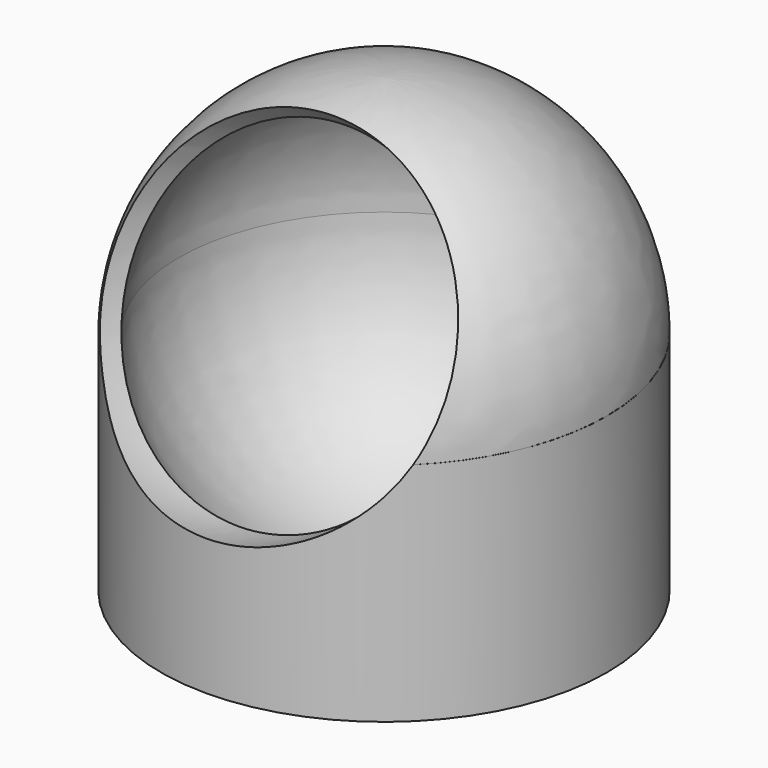
from build123d import *

# Parameters (mm, degrees)
F4_R     = 25.2
F7_DEPTH = 25.4980942398


with BuildPart() as f2:
    # F1 (on Front) → F2 (revolve)
    with BuildSketch(Plane.XZ):
        with BuildLine():
            ThreePointArc((0, 0), (17.8293562003, 7.5774317225), (25.1882466714, 25.4980942398))
            ThreePointArc((25.1882466714, 25.4980942398), (17.8293562003, 43.4187567571), (0, 50.9961884796))
            Line((0, 50.9961884796), (0, 48.9960262735))
            ThreePointArc((0, 48.9960262735), (16.4151143283, 42.0045141541), (23.1882466714, 25.4980942398))
            ThreePointArc((23.1882466714, 25.4980942398), (16.4151143283, 8.9916743255), (0, 2.0001622061))
            Line((0, 2.0001622061), (0, 0))
        make_face()
        with BuildLine():
            ThreePointArc((23.1882466714, 25.4980942398), (16.4151143283, 42.0045141541), (0, 48.9960262735))
            Line((0, 48.9960262735), (0, 2.0001622061))
            ThreePointArc((0, 2.0001622061), (16.4151143283, 8.9916743255), (23.1882466714, 25.4980942398))
        make_face()
    revolve(axis=Axis((0, 0, 25.4980942398), (0, 0, -1)))

    # F4 (on Top) → F7 (join, through all)
    with BuildSketch(Plane.XY):
        Circle(F4_R)
    extrude(amount=F7_DEPTH)


with BuildPart() as f3:
    # F1 (on Front) → F3 (revolve)
    with BuildSketch(Plane.XZ):
        with BuildLine():
            ThreePointArc((23.1882466714, 25.4980942398), (16.4151143283, 42.0045141541), (0, 48.9960262735))
            Line((0, 48.9960262735), (0, 2.0001622061))
            ThreePointArc((0, 2.0001622061), (16.4151143283, 8.9916743255), (23.1882466714, 25.4980942398))
        make_face()
    revolve(axis=Axis((0, 0, 25.4980942398), (0, 0, -1)))


with BuildPart() as f9:
    # F8 (on Right) → F9 (revolve)
    with BuildSketch(Plane.YZ):
        with BuildLine():
            Line((-19.8910422623, 14.6723976359), (-19.8910422623, 54.6723976359))
            ThreePointArc((-19.8910422623, 54.6723976359), (-39.8910422623, 34.6723976359), (-19.8910422623, 14.6723976359))
        make_face()
    revolve(axis=Axis((0, -19.8910422623, 34.6723976359), (0, 0, -1)))


with BuildPart() as f2_1:
    add(f2.part)

    # F10: cut F9
    add(f9.part, mode=Mode.SUBTRACT)

    # F11: cut F3
    add(f3.part, mode=Mode.SUBTRACT)


solid = f2_1.part
